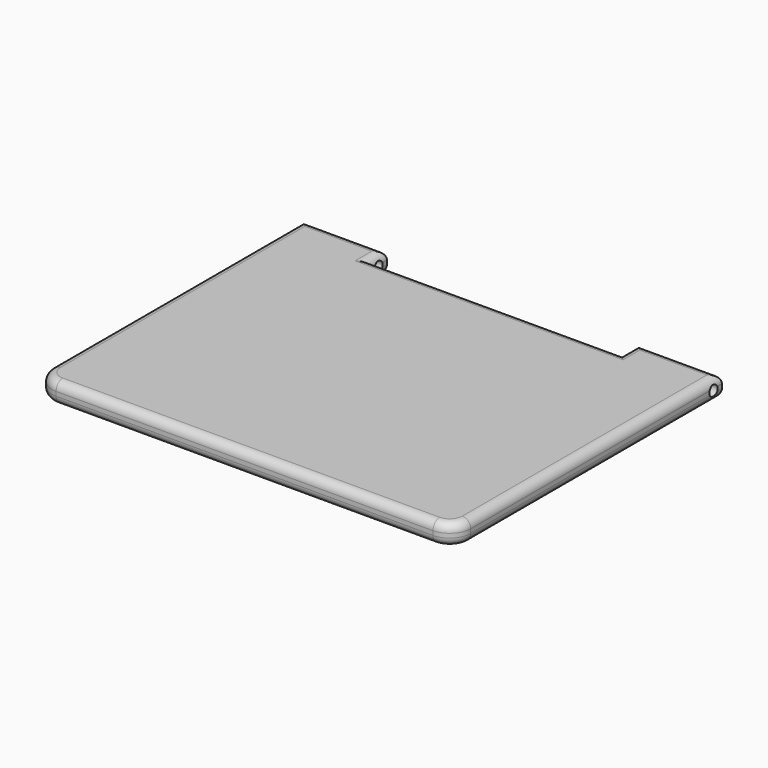
from build123d import *

# Parameters (mm, degrees)
F0_W         = 254
F0_H         = 203.2
F1_DEPTH     = 12.7
F4_DEPTH     = 254.001
F2_W         = 76.2
F2_H         = 12.7
F5_DEPTH     = 12.701
F6_T1_DEPTH  = 228.6
F6_T3_DEPTH  = 279.4
F6_T5_DEPTH  = 76.2
F6_T7_DEPTH  = 25.4
F6_T9_DEPTH  = 152.4
F6_T11_DEPTH = 76.2
F6_T17_DEPTH = 38.1
F6_T21_DEPTH = 165.1
F6_T28_DEPTH = 38.1
F6_T32_DEPTH = 165.1
F6_T39_DEPTH = 38.1
F6_T43_DEPTH = 165.1
F6_T50_DEPTH = 165.1
F6_T54_DEPTH = 38.1
F7_T1_DEPTH  = 12.7000000002
F7_T4_ANGLE  = 90
F7_T6_ANGLE  = 90
F7_T8_ANGLE  = 90
F7_T10_ANGLE = 90


# Not quite as in the source:
# - a fillet or chamfer that OpenCascade refuses, or shapes differently, is made with other operations: its cross-section is extruded or revolved along the edge and cut away or added


with BuildPart() as f1:
    # F0 (on Top) → F1 (new body)
    with BuildSketch(Plane.XY):
        Rectangle(F0_W, F0_H)
    extrude(amount=F1_DEPTH)

    # F3 (on face) → F4 (cut, through all)
    with BuildSketch(Plane(origin=(-127, 0, 0), x_dir=(0, -1, 0), z_dir=(-1, 0, 0))):
        with BuildLine():
            ThreePointArc((-92.075, 6.35), (-95.25, 9.525), (-98.425, 6.35))
            Line((-98.425, 6.35), (-92.075, 6.35))
        make_face()
        with BuildLine():
            Line((-92.075, 6.35), (-98.425, 6.35))
            ThreePointArc((-98.425, 6.35), (-95.25, 3.175), (-92.075, 6.35))
        make_face()
    extrude(amount=-F4_DEPTH, mode=Mode.SUBTRACT)

    # F2 (on face) → F5 (cut, through all)
    with BuildSketch(Plane.XY.offset(12.7)):
        with Locations((-38.1, 95.25)):
            Rectangle(F2_W, F2_H)
        with Locations((38.1, 95.25)):
            Rectangle(F2_W, F2_H)
    extrude(amount=-F5_DEPTH, mode=Mode.SUBTRACT)

    # F6: fillet of radius 5.08 on 16 edges, made by hand

    # F6_s2 → F6_t1 (cut)
    with BuildSketch(Plane.XZ.offset(-114.3)):
        with BuildLine():
            ThreePointArc((121.92, 12.7), (125.5121024484, 11.2121024484), (127, 7.62))
            Line((127, 7.62), (127, 12.7))
            Line((127, 12.7), (121.92, 12.7))
        make_face()
        with BuildLine():
            ThreePointArc((-121.92, 12.7), (-125.5121024484, 11.2121024484), (-127, 7.62))
            Line((-127, 7.62), (-127, 12.7))
            Line((-127, 12.7), (-121.92, 12.7))
        make_face()
        with BuildLine():
            ThreePointArc((121.92, 0), (125.5121024484, 1.4878975516), (127, 5.08))
            Line((127, 5.08), (127, 0))
            Line((127, 0), (121.92, 0))
        make_face()
        with BuildLine():
            ThreePointArc((-121.92, 0), (-125.5121024484, 1.4878975516), (-127, 5.08))
            Line((-127, 5.08), (-127, 0))
            Line((-127, 0), (-121.92, 0))
        make_face()
    extrude(amount=F6_T1_DEPTH, mode=Mode.SUBTRACT)

    # F6_s4 → F6_t3 (cut)
    with BuildSketch(Plane.YZ.offset(-139.7)):
        with BuildLine():
            ThreePointArc((-96.52, 12.7), (-100.1121024484, 11.2121024484), (-101.6, 7.62))
            Line((-101.6, 7.62), (-101.6, 12.7))
            Line((-101.6, 12.7), (-96.52, 12.7))
        make_face()
        with BuildLine():
            ThreePointArc((-96.52, 0), (-100.1121024484, 1.4878975516), (-101.6, 5.08))
            Line((-101.6, 5.08), (-101.6, 0))
            Line((-101.6, 0), (-96.52, 0))
        make_face()
    extrude(amount=F6_T3_DEPTH, mode=Mode.SUBTRACT)

    # F6_s6 → F6_t5 (cut)
    with BuildSketch(Plane.YZ.offset(-139.7)):
        with BuildLine():
            ThreePointArc((96.52, 12.7), (100.1121024484, 11.2121024484), (101.6, 7.62))
            Line((101.6, 7.62), (101.6, 12.7))
            Line((101.6, 12.7), (96.52, 12.7))
        make_face()
        with BuildLine():
            ThreePointArc((96.52, 0), (100.1121024484, 1.4878975516), (101.6, 5.08))
            Line((101.6, 5.08), (101.6, 0))
            Line((101.6, 0), (96.52, 0))
        make_face()
    extrude(amount=F6_T5_DEPTH, mode=Mode.SUBTRACT)

    # F6_s8 → F6_t7 (cut)
    with BuildSketch(Plane.XZ.offset(-114.3)):
        with BuildLine():
            ThreePointArc((-81.28, 12.7), (-77.6878975516, 11.2121024484), (-76.2, 7.62))
            Line((-76.2, 7.62), (-76.2, 12.7))
            Line((-76.2, 12.7), (-81.28, 12.7))
        make_face()
        with BuildLine():
            ThreePointArc((76.2, 7.62), (77.6878975516, 11.2121024484), (81.28, 12.7))
            Line((81.28, 12.7), (76.2, 12.7))
            Line((76.2, 12.7), (76.2, 7.62))
        make_face()
        with BuildLine():
            ThreePointArc((-81.28, 0), (-77.6878975516, 1.4878975516), (-76.2, 5.08))
            Line((-76.2, 5.08), (-76.2, 0))
            Line((-76.2, 0), (-81.28, 0))
        make_face()
        with BuildLine():
            ThreePointArc((81.28, 0), (77.6878975516, 1.4878975516), (76.2, 5.08))
            Line((76.2, 5.08), (76.2, 0))
            Line((76.2, 0), (81.28, 0))
        make_face()
    extrude(amount=F6_T7_DEPTH, mode=Mode.SUBTRACT)

    # F6_s10 → F6_t9 (cut)
    with BuildSketch(Plane.YZ.offset(-76.2)):
        with BuildLine():
            ThreePointArc((83.82, 12.7), (87.4121024484, 11.2121024484), (88.9, 7.62))
            Line((88.9, 7.62), (88.9, 12.7))
            Line((88.9, 12.7), (83.82, 12.7))
        make_face()
        with BuildLine():
            ThreePointArc((83.82, 0), (87.4121024484, 1.4878975516), (88.9, 5.08))
            Line((88.9, 5.08), (88.9, 0))
            Line((88.9, 0), (83.82, 0))
        make_face()
    extrude(amount=F6_T9_DEPTH, mode=Mode.SUBTRACT)

    # F6_s12 → F6_t11 (cut)
    with BuildSketch(Plane.YZ.offset(63.5)):
        with BuildLine():
            ThreePointArc((101.6, 7.62), (100.1121024484, 11.2121024484), (96.52, 12.7))
            Line((96.52, 12.7), (101.6, 12.7))
            Line((101.6, 12.7), (101.6, 7.62))
        make_face()
        with BuildLine():
            ThreePointArc((101.6, 5.08), (100.1121024484, 1.4878975516), (96.52, 0))
            Line((96.52, 0), (101.6, 0))
            Line((101.6, 0), (101.6, 5.08))
        make_face()
    extrude(amount=F6_T11_DEPTH, mode=Mode.SUBTRACT)


with BuildPart() as f6_tool15:
    # F6_s16 → F6_t17 (new body)
    with BuildSketch(Plane.XZ.offset(-114.3)):
        with BuildLine():
            ThreePointArc((-81.28, 12.7), (-77.6878975516, 11.2121024484), (-76.2, 7.62))
            Line((-76.2, 7.62), (-76.2, 12.7))
            Line((-76.2, 12.7), (-81.28, 12.7))
        make_face()
    extrude(amount=F6_T17_DEPTH)

    split(bisect_by=Plane.XZ.offset(-88.9), keep=Keep.TOP)


with BuildPart() as f6_tool19:
    # F6_s20 → F6_t21 (new body)
    with BuildSketch(Plane.YZ.offset(-88.9)):
        with BuildLine():
            ThreePointArc((83.82, 12.7), (87.4121024484, 11.2121024484), (88.9, 7.62))
            Line((88.9, 7.62), (88.9, 12.7))
            Line((88.9, 12.7), (83.82, 12.7))
        make_face()
    extrude(amount=F6_T21_DEPTH)

    split(bisect_by=Plane.YZ.offset(-76.2), keep=Keep.BOTTOM)


with BuildPart() as f6_tool15_1:
    add(f6_tool15.part)

    # F6_t23: intersect F6_tool19
    add(f6_tool19.part, mode=Mode.INTERSECT)


with BuildPart() as f1_1:
    add(f1.part)

    # F6_t13: cut F6_tool15
    add(f6_tool15_1.part, mode=Mode.SUBTRACT)


with BuildPart() as f6_tool26:
    # F6_s27 → F6_t28 (new body)
    with BuildSketch(Plane.XZ.offset(-76.2)):
        with BuildLine():
            ThreePointArc((76.2, 7.62), (77.6878975516, 11.2121024484), (81.28, 12.7))
            Line((81.28, 12.7), (76.2, 12.7))
            Line((76.2, 12.7), (76.2, 7.62))
        make_face()
    extrude(amount=-F6_T28_DEPTH)

    split(bisect_by=Plane.XZ.offset(-88.9), keep=Keep.TOP)


with BuildPart() as f6_tool30:
    # F6_s31 → F6_t32 (new body)
    with BuildSketch(Plane.YZ.offset(-76.2)):
        with BuildLine():
            ThreePointArc((83.82, 12.7), (87.4121024484, 11.2121024484), (88.9, 7.62))
            Line((88.9, 7.62), (88.9, 12.7))
            Line((88.9, 12.7), (83.82, 12.7))
        make_face()
    extrude(amount=F6_T32_DEPTH)

    split(bisect_by=Plane.YZ.offset(76.2), keep=Keep.TOP)


with BuildPart() as f6_tool26_1:
    add(f6_tool26.part)

    # F6_t34: intersect F6_tool30
    add(f6_tool30.part, mode=Mode.INTERSECT)


with BuildPart() as f1_2:
    add(f1_1.part)

    # F6_t24: cut F6_tool26
    add(f6_tool26_1.part, mode=Mode.SUBTRACT)


with BuildPart() as f6_tool37:
    # F6_s38 → F6_t39 (new body)
    with BuildSketch(Plane.XZ.offset(-114.3)):
        with BuildLine():
            ThreePointArc((-81.28, 0), (-77.6878975516, 1.4878975516), (-76.2, 5.08))
            Line((-76.2, 5.08), (-76.2, 0))
            Line((-76.2, 0), (-81.28, 0))
        make_face()
    extrude(amount=F6_T39_DEPTH)

    split(bisect_by=Plane.XZ.offset(-88.9), keep=Keep.TOP)


with BuildPart() as f6_tool41:
    # F6_s42 → F6_t43 (new body)
    with BuildSketch(Plane.YZ.offset(-88.9)):
        with BuildLine():
            ThreePointArc((83.82, 0), (87.4121024484, 1.4878975516), (88.9, 5.08))
            Line((88.9, 5.08), (88.9, 0))
            Line((88.9, 0), (83.82, 0))
        make_face()
    extrude(amount=F6_T43_DEPTH)

    split(bisect_by=Plane.YZ.offset(-76.2), keep=Keep.BOTTOM)


with BuildPart() as f6_tool37_1:
    add(f6_tool37.part)

    # F6_t45: intersect F6_tool41
    add(f6_tool41.part, mode=Mode.INTERSECT)


with BuildPart() as f1_3:
    add(f1_2.part)

    # F6_t35: cut F6_tool37
    add(f6_tool37_1.part, mode=Mode.SUBTRACT)


with BuildPart() as f6_tool48:
    # F6_s49 → F6_t50 (new body)
    with BuildSketch(Plane.YZ.offset(-76.2)):
        with BuildLine():
            ThreePointArc((83.82, 0), (87.4121024484, 1.4878975516), (88.9, 5.08))
            Line((88.9, 5.08), (88.9, 0))
            Line((88.9, 0), (83.82, 0))
        make_face()
    extrude(amount=F6_T50_DEPTH)

    split(bisect_by=Plane.YZ.offset(76.2), keep=Keep.TOP)


with BuildPart() as f6_tool52:
    # F6_s53 → F6_t54 (new body)
    with BuildSketch(Plane.XZ.offset(-76.2)):
        with BuildLine():
            ThreePointArc((81.28, 0), (77.6878975516, 1.4878975516), (76.2, 5.08))
            Line((76.2, 5.08), (76.2, 0))
            Line((76.2, 0), (81.28, 0))
        make_face()
    extrude(amount=-F6_T54_DEPTH)

    split(bisect_by=Plane.XZ.offset(-88.9), keep=Keep.TOP)


with BuildPart() as f6_tool48_1:
    add(f6_tool48.part)

    # F6_t56: intersect F6_tool52
    add(f6_tool52.part, mode=Mode.INTERSECT)


with BuildPart() as f1_4:
    add(f1_3.part)

    # F6_t46: cut F6_tool48
    add(f6_tool48_1.part, mode=Mode.SUBTRACT)

    # F7: fillet of radius 12.7 on 2 edges, made by hand

    # F7_s2 → F7_t1 (cut)
    with BuildSketch(Plane.XY):
        with BuildLine():
            ThreePointArc((-114.3, -101.6), (-123.2802561211, -97.8802561211), (-127, -88.9))
            Line((-127, -88.9), (-127, -101.6))
            Line((-127, -101.6), (-114.3, -101.6))
        make_face()
        with BuildLine():
            ThreePointArc((114.3, -101.6), (123.2802561211, -97.8802561211), (127, -88.9))
            Line((127, -88.9), (127, -101.6))
            Line((127, -101.6), (114.3, -101.6))
        make_face()
    extrude(amount=F7_T1_DEPTH, mode=Mode.SUBTRACT)

    # F7_s3 → F7_t4 (revolve, cut)
    with BuildSketch(Plane.XZ.offset(88.9)):
        with BuildLine():
            ThreePointArc((121.9199999999, 0), (125.5121024484, 1.4878975516), (127, 5.0800000001))
            Line((127, 5.0800000001), (127, 0))
            Line((127, 0), (121.9199999999, 0))
        make_face()
    revolve(axis=Axis((114.3, -88.9, 0), (0, 0, -1)), revolution_arc=F7_T4_ANGLE, mode=Mode.SUBTRACT)

    # F7_s5 → F7_t6 (revolve, cut)
    with BuildSketch(Plane.YZ.offset(114.3)):
        with BuildLine():
            ThreePointArc((-96.5199999999, 12.7), (-100.1121024484, 11.2121024484), (-101.6, 7.6199999999))
            Line((-101.6, 7.6199999999), (-101.6, 12.7))
            Line((-101.6, 12.7), (-96.5199999999, 12.7))
        make_face()
    revolve(axis=Axis((114.3, -88.9, 12.7), (0, 0, 1)), revolution_arc=F7_T6_ANGLE, mode=Mode.SUBTRACT)

    # F7_s7 → F7_t8 (revolve, cut)
    with BuildSketch(Plane.YZ.offset(-114.3)):
        with BuildLine():
            ThreePointArc((-96.5199999999, 0), (-100.1121024484, 1.4878975516), (-101.6, 5.0800000001))
            Line((-101.6, 5.0800000001), (-101.6, 0))
            Line((-101.6, 0), (-96.5199999999, 0))
        make_face()
    revolve(axis=Axis((-114.3, -88.9, 0), (0, 0, -1)), revolution_arc=F7_T8_ANGLE, mode=Mode.SUBTRACT)

    # F7_s9 → F7_t10 (revolve, cut)
    with BuildSketch(Plane.XZ.offset(88.9)):
        with BuildLine():
            ThreePointArc((-121.9199999999, 12.7), (-125.5121024484, 11.2121024484), (-127, 7.6199999999))
            Line((-127, 7.6199999999), (-127, 12.7))
            Line((-127, 12.7), (-121.9199999999, 12.7))
        make_face()
    revolve(axis=Axis((-114.3, -88.9, 12.7), (0, 0, 1)), revolution_arc=F7_T10_ANGLE, mode=Mode.SUBTRACT)


solid = f1_4.part
